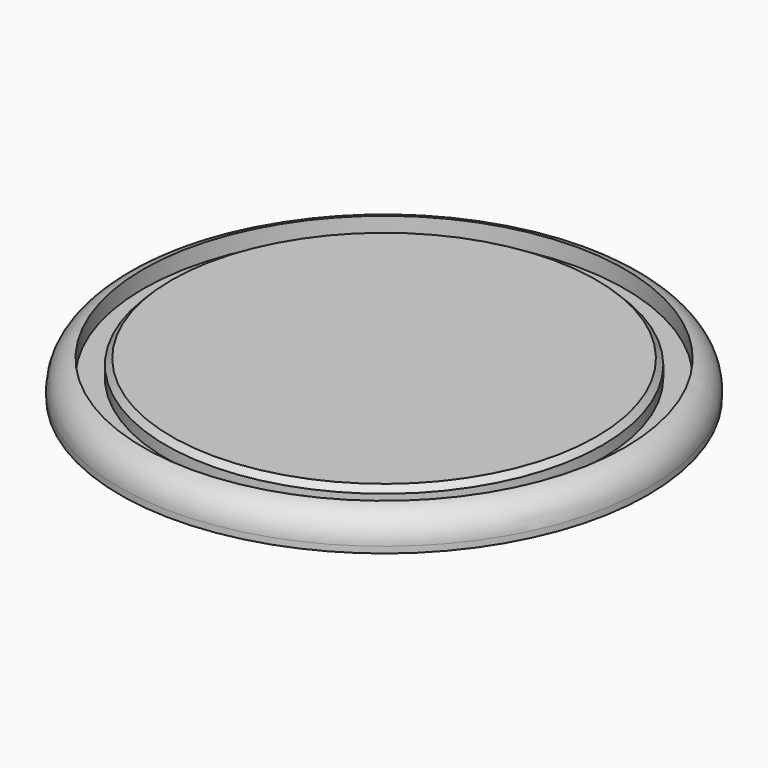
from build123d import *

# Parameters (mm, degrees)
F0_R     = 46
F0_R_2   = 42
F0_R_3   = 38
F1_DEPTH = 3
F2_DEPTH = 6
F4_SIZE  = 1


# Not quite as in the source:
# - a fillet or chamfer that OpenCascade refuses, or shapes differently, is made with other operations: its cross-section is extruded or revolved along the edge and cut away or added


with BuildPart() as f1:
    # F0 (on Top) → F1 (new body)
    with BuildSketch(Plane.XY):
        Circle(F0_R)
        Circle(F0_R_2, mode=Mode.SUBTRACT)
        Circle(F0_R_2)
        Circle(F0_R_3, mode=Mode.SUBTRACT)
        Circle(F0_R_3)
    extrude(amount=F1_DEPTH)

    # F0 (on Top) → F2 (join)
    with BuildSketch(Plane.XY):
        Circle(F0_R)
        Circle(F0_R_2, mode=Mode.SUBTRACT)
        Circle(F0_R_3)
    extrude(amount=F2_DEPTH)

    # F3: fillet of radius 5 on 1 edges, made by hand

    # F3_s1 → F3_t2 (revolve, cut)
    with BuildSketch(Plane.XZ):
        with BuildLine():
            ThreePointArc((46, 1.1010205144), (44.8729833462, 4.2632981746), (42, 6))
            Line((42, 6), (46, 6))
            Line((46, 6), (46, 1.1010205144))
        make_face()
    revolve(axis=Axis((0, 0, 6), (0, 0, 1)), mode=Mode.SUBTRACT)

    # F4
    f4_edges = [f1.edges().sort_by_distance(p)[0] for p in [
        (-38, 0, 6),
    ]]
    chamfer(f4_edges, length=F4_SIZE)


solid = f1.part
